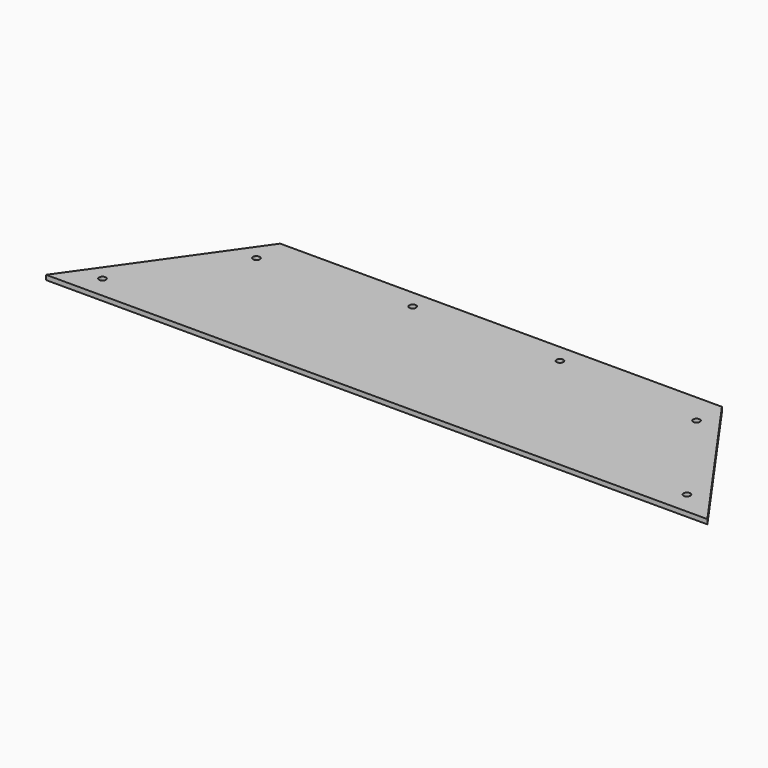
from build123d import *

# Parameters (mm, degrees)
F0_R     = 2.3114
F1_DEPTH = 3.175


with BuildPart() as f1:
    # F0 (on Top) → F1 (new body)
    with BuildSketch(Plane.XY):
        with BuildLine():
            Line((-451.5609132883, 3.4527331373), (-420.9521720122, 3.4527331373))
            Line((-420.9521720122, 3.4527331373), (-359.0199119076, 91.1230753634))
            Line((-359.0199119076, 91.1230753634), (-379.4389155629, 105.5475091382))
            Line((-379.4389155629, 105.5475091382), (-386.6511324503, 95.3380073106))
            Line((-386.6511324503, 95.3380073106), (-378.3294900246, 89.4594158723))
            ThreePointArc((-378.3294900246, 89.4594158723), (-375.7419979554, 90.3287620732), (-374.1302306227, 88.1257904232))
            ThreePointArc((-374.1302306227, 88.1257904232), (-375.3786094336, 86.0733392273), (-377.7752560717, 86.2379310212))
            Line((-377.7752560717, 86.2379310212), (-424.151080008, 20.5890373971))
            ThreePointArc((-424.151080008, 20.5890373971), (-423.4322542612, 19.7641991843), (-423.1733054571, 18.7011779952))
            ThreePointArc((-423.1733054571, 18.7011779952), (-426.1843381244, 16.4982063451), (-427.3725648591, 20.0348034442))
            Line((-427.3725648591, 20.0348034442), (-435.6942072848, 25.9133948826))
            Line((-435.6942072848, 25.9133948826), (-451.5609132883, 3.4527331373))
        make_face()
        Polygon((-359.0199119076, 91.1230753634), (-420.9521720122, 3.4527331373), (-2.4390867117, 3.4527331373), (-77, 109), (-177, 109), (-227, 109), (-277, 109), (-377, 109), (-379.4389155629, 105.5475091382), align=None)
        with Locations((-28.5152945429, 18.7011779952)):
            Circle(F0_R, mode=Mode.SUBTRACT)
        with BuildLine():
            ThreePointArc((-274.6886, 96.5), (-278.634406614, 94.865593386), (-277, 98.8114))
            ThreePointArc((-277, 98.8114), (-275.365593386, 98.134406614), (-274.6886, 96.5))
        make_face(mode=Mode.SUBTRACT)
        with Locations((-77.5583693773, 88.1257904232)):
            Circle(F0_R, mode=Mode.SUBTRACT)
        with BuildLine():
            ThreePointArc((-174.6886, 96.5), (-177, 94.1886), (-179.3114, 96.5))
            ThreePointArc((-179.3114, 96.5), (-178.634406614, 98.134406614), (-177, 98.8114))
            ThreePointArc((-177, 98.8114), (-175.365593386, 98.134406614), (-174.6886, 96.5))
        make_face(mode=Mode.SUBTRACT)
        with BuildLine():
            Line((-415.5, 54.5), (-435.6942072848, 25.9133948826))
            Line((-435.6942072848, 25.9133948826), (-427.3725648591, 20.0348034442))
            ThreePointArc((-427.3725648591, 20.0348034442), (-425.8766080436, 20.9791117788), (-424.151080008, 20.5890373971))
            Line((-424.151080008, 20.5890373971), (-377.7752560717, 86.2379310212))
            ThreePointArc((-377.7752560717, 86.2379310212), (-378.7195644063, 87.7338878367), (-378.3294900246, 89.4594158723))
            Line((-378.3294900246, 89.4594158723), (-386.6511324503, 95.3380073106))
            Line((-386.6511324503, 95.3380073106), (-415.5, 54.5))
        make_face()
    extrude(amount=F1_DEPTH)


solid = f1.part
